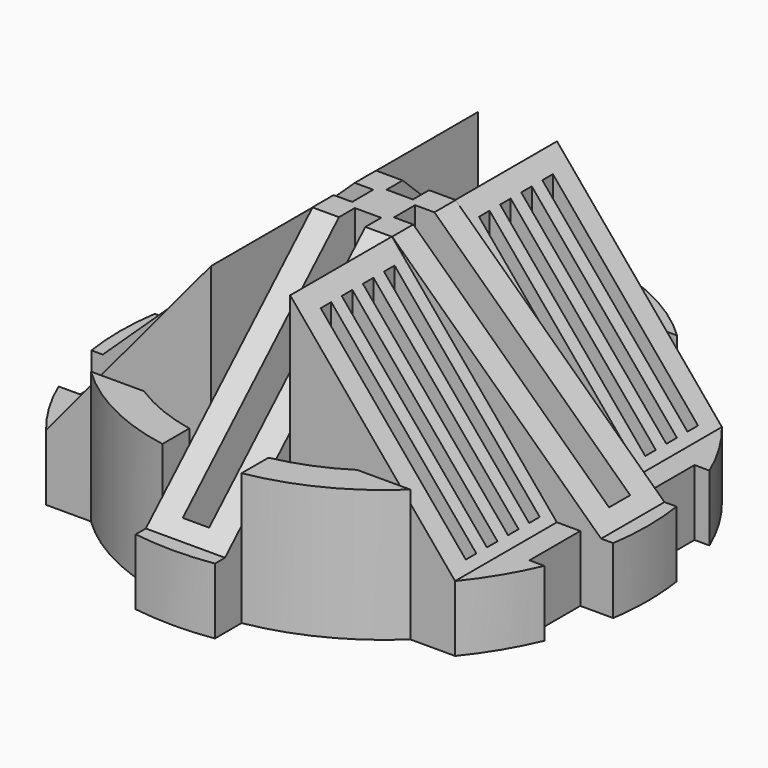
from build123d import *

# Parameters (mm, degrees)
F2_DEPTH  = 12.7
F3_DEPTH  = 25.4
F4_DEPTH  = 38.1
F5_DEPTH  = 50.8
F6_DEPTH  = 50.8
F7_DEPTH  = 50.8
F11_DEPTH = 15.24
F12_DEPTH = 15.24
F13_DEPTH = 15.24
F15_DEPTH = 15.24
F16_W     = 41.402
F16_H     = 5.08
F16_W_2   = 5.08
F16_H_2   = 41.402
F17_DEPTH = 44.45
F18_DEPTH = 50.8
F21_DEPTH = 24.4856
F19_W     = 27.94
F19_H     = 2.54
F22_DEPTH = 44.45
F24_DEPTH = 24.4856
F26_DEPTH = 24.4856
F28_DEPTH = 24.4856
F29_DEPTH = 50.801
F30_DEPTH = 25.4


# Not quite as in the source:
# - after a boolean that leaves OpenCascade's solid faulty, fix() repairs it
# - a feature names something its author has since deleted; it is built from what else it names


with BuildPart() as f2:
    # F1 (on Top) → F2 (new body)
    with BuildSketch(Plane.XY):
        with BuildLine():
            ThreePointArc((50.2252486305, -7.62), (50.6561083702, -3.8208225272), (50.8, 0))
            ThreePointArc((50.8, 0), (50.6561083702, 3.8208225272), (50.2252486305, 7.62))
            Line((50.2252486305, 7.62), (43.8856464383, 7.62))
            Line((43.8856464383, 7.62), (43.8856464383, -7.62))
            Line((43.8856464383, -7.62), (50.2252486305, -7.62))
        make_face()
        with BuildLine():
            Line((43.8856464383, 7.62), (50.2252486305, 7.62))
            ThreePointArc((50.2252486305, 7.62), (48.8754001329, 13.850460709), (46.7558464383, 19.8628))
            Line((46.7558464383, 19.8628), (43.8856464383, 19.8628))
            Line((43.8856464383, 19.8628), (43.8856464383, 7.62))
        make_face()
        with BuildLine():
            ThreePointArc((46.7558464383, -19.8628), (48.8754001329, -13.850460709), (50.2252486305, -7.62))
            Line((50.2252486305, -7.62), (43.8856464383, -7.62))
            Line((43.8856464383, -7.62), (43.8856464383, -19.8628))
            Line((43.8856464383, -19.8628), (46.7558464383, -19.8628))
        make_face()
        with BuildLine():
            Line((43.8856464383, 19.8628), (46.7558464383, 19.8628))
            ThreePointArc((46.7558464383, 19.8628), (43.4950311771, 26.2454236564), (39.3683940318, 32.1056))
            Line((39.3683940318, 32.1056), (30.7413882029, 32.1056))
            ThreePointArc((30.7413882029, 32.1056), (35.7808122406, 26.3730160468), (39.7652068542, 19.8628))
            Line((39.7652068542, 19.8628), (43.8856464383, 19.8628))
        make_face()
        with BuildLine():
            ThreePointArc((39.3683940318, -32.1056), (43.4950311771, -26.2454236564), (46.7558464383, -19.8628))
            Line((46.7558464383, -19.8628), (43.8856464383, -19.8628))
            Line((43.8856464383, -19.8628), (39.7652068542, -19.8628))
            ThreePointArc((39.7652068542, -19.8628), (35.7808122406, -26.3730160468), (30.7413882029, -32.1056))
            Line((30.7413882029, -32.1056), (39.3683940318, -32.1056))
        make_face()
        with BuildLine():
            Line((30.7413882029, 32.1056), (39.3683940318, 32.1056))
            ThreePointArc((39.3683940318, 32.1056), (25.1805025773, 44.1200894146), (7.62, 50.2252486305))
            Line((7.62, 50.2252486305), (7.62, 43.7919867099))
            ThreePointArc((7.62, 43.7919867099), (20.0509833873, 39.670651182), (30.7413882029, 32.1056))
        make_face()
        with BuildLine():
            ThreePointArc((7.62, -50.2252486305), (25.1805025773, -44.1200894146), (39.3683940318, -32.1056))
            Line((39.3683940318, -32.1056), (30.7413882029, -32.1056))
            ThreePointArc((30.7413882029, -32.1056), (20.0509833873, -39.670651182), (7.62, -43.7919867099))
            Line((7.62, -43.7919867099), (7.62, -50.2252486305))
        make_face()
        with BuildLine():
            Line((7.62, 43.7919867099), (7.62, 50.2252486305))
            ThreePointArc((7.62, 50.2252486305), (0, 50.8), (-7.62, 50.2252486305))
            Line((-7.62, 50.2252486305), (-7.62, 43.7919867099))
            ThreePointArc((-7.62, 43.7919867099), (0, 44.45), (7.62, 43.7919867099))
        make_face()
        with BuildLine():
            Line((20.5143961315, 32.1056), (30.7413882029, 32.1056))
            ThreePointArc((30.7413882029, 32.1056), (20.0509833873, 39.670651182), (7.62, 43.7919867099))
            Line((7.62, 43.7919867099), (7.62, 37.33022368))
            ThreePointArc((7.62, 37.33022368), (14.3076984372, 35.3114679025), (20.5143961315, 32.1056))
        make_face()
        with BuildLine():
            ThreePointArc((-7.62, -50.2252486305), (0, -50.8), (7.62, -50.2252486305))
            Line((7.62, -50.2252486305), (7.62, -43.7919867099))
            ThreePointArc((7.62, -43.7919867099), (0, -44.45), (-7.62, -43.7919867099))
            Line((-7.62, -43.7919867099), (-7.62, -50.2252486305))
        make_face()
        with BuildLine():
            ThreePointArc((7.62, -43.7919867099), (20.0509833873, -39.670651182), (30.7413882029, -32.1056))
            Line((30.7413882029, -32.1056), (20.5143961315, -32.1056))
            ThreePointArc((20.5143961315, -32.1056), (14.3076984372, -35.3114679025), (7.62, -37.33022368))
            Line((7.62, -37.33022368), (7.62, -43.7919867099))
        make_face()
        with BuildLine():
            Line((-7.62, 43.7919867099), (-7.62, 50.2252486305))
            ThreePointArc((-7.62, 50.2252486305), (-25.1805025773, 44.1200894146), (-39.3683940318, 32.1056))
            Line((-39.3683940318, 32.1056), (-30.7413882029, 32.1056))
            ThreePointArc((-30.7413882029, 32.1056), (-20.0509833873, 39.670651182), (-7.62, 43.7919867099))
        make_face()
        with BuildLine():
            ThreePointArc((-39.3683940318, -32.1056), (-25.1805025773, -44.1200894146), (-7.62, -50.2252486305))
            Line((-7.62, -50.2252486305), (-7.62, -43.7919867099))
            ThreePointArc((-7.62, -43.7919867099), (-20.0509833873, -39.670651182), (-30.7413882029, -32.1056))
            Line((-30.7413882029, -32.1056), (-39.3683940318, -32.1056))
        make_face()
        with BuildLine():
            Line((-30.7413882029, 32.1056), (-39.3683940318, 32.1056))
            ThreePointArc((-39.3683940318, 32.1056), (-43.4950311771, 26.2454236564), (-46.7558464383, 19.8628))
            Line((-46.7558464383, 19.8628), (-42.6407977939, 19.8628))
            Line((-42.6407977939, 19.8628), (-39.7652068542, 19.8628))
            ThreePointArc((-39.7652068542, 19.8628), (-35.7808122406, 26.3730160468), (-30.7413882029, 32.1056))
        make_face()
        with BuildLine():
            Line((-7.62, 37.33022368), (-7.62, 43.7919867099))
            ThreePointArc((-7.62, 43.7919867099), (-20.0509833873, 39.670651182), (-30.7413882029, 32.1056))
            Line((-30.7413882029, 32.1056), (-20.5143961315, 32.1056))
            ThreePointArc((-20.5143961315, 32.1056), (-14.3076984372, 35.3114679025), (-7.62, 37.33022368))
        make_face()
        with BuildLine():
            ThreePointArc((-46.7558464383, -19.8628), (-43.4950311771, -26.2454236564), (-39.3683940318, -32.1056))
            Line((-39.3683940318, -32.1056), (-30.7413882029, -32.1056))
            ThreePointArc((-30.7413882029, -32.1056), (-35.7808122406, -26.3730160468), (-39.7652068542, -19.8628))
            Line((-39.7652068542, -19.8628), (-42.6407977939, -19.8628))
            Line((-42.6407977939, -19.8628), (-46.7558464383, -19.8628))
        make_face()
        with BuildLine():
            ThreePointArc((-30.7413882029, -32.1056), (-20.0509833873, -39.670651182), (-7.62, -43.7919867099))
            Line((-7.62, -43.7919867099), (-7.62, -37.33022368))
            ThreePointArc((-7.62, -37.33022368), (-14.2009349705, -35.3545392554), (-20.32, -32.2289869527))
            ThreePointArc((-20.32, -32.2289869527), (-20.4172912734, -32.1674403249), (-20.5143961315, -32.1056))
            Line((-20.5143961315, -32.1056), (-30.7413882029, -32.1056))
        make_face()
        with BuildLine():
            Line((-42.6407977939, 19.8628), (-46.7558464383, 19.8628))
            ThreePointArc((-46.7558464383, 19.8628), (-48.8754001329, 13.850460709), (-50.2252486305, 7.62))
            Line((-50.2252486305, 7.62), (-42.6407977939, 7.62))
            Line((-42.6407977939, 7.62), (-42.6407977939, 19.8628))
        make_face()
        with BuildLine():
            ThreePointArc((-50.2252486305, -7.62), (-48.8754001329, -13.850460709), (-46.7558464383, -19.8628))
            Line((-46.7558464383, -19.8628), (-42.6407977939, -19.8628))
            Line((-42.6407977939, -19.8628), (-42.6407977939, -7.62))
            Line((-42.6407977939, -7.62), (-50.2252486305, -7.62))
        make_face()
        with BuildLine():
            Line((-42.6407977939, 7.62), (-50.2252486305, 7.62))
            ThreePointArc((-50.2252486305, 7.62), (-50.8, 0), (-50.2252486305, -7.62))
            Line((-50.2252486305, -7.62), (-42.6407977939, -7.62))
            Line((-42.6407977939, -7.62), (-42.6407977939, 7.62))
        make_face()
    extrude(amount=F2_DEPTH)

    # F1 (on Top) → F3 (join)
    with BuildSketch(Plane.XY):
        with BuildLine():
            ThreePointArc((-30.7413882029, -32.1056), (-20.0509833873, -39.670651182), (-7.62, -43.7919867099))
            Line((-7.62, -43.7919867099), (-7.62, -37.33022368))
            ThreePointArc((-7.62, -37.33022368), (-14.2009349705, -35.3545392554), (-20.32, -32.2289869527))
            ThreePointArc((-20.32, -32.2289869527), (-20.4172912734, -32.1674403249), (-20.5143961315, -32.1056))
            Line((-20.5143961315, -32.1056), (-30.7413882029, -32.1056))
        make_face()
        with BuildLine():
            ThreePointArc((7.62, -43.7919867099), (20.0509833873, -39.670651182), (30.7413882029, -32.1056))
            Line((30.7413882029, -32.1056), (20.5143961315, -32.1056))
            ThreePointArc((20.5143961315, -32.1056), (14.3076984372, -35.3114679025), (7.62, -37.33022368))
            Line((7.62, -37.33022368), (7.62, -43.7919867099))
        make_face()
        with BuildLine():
            Line((20.5143961315, -32.1056), (30.7413882029, -32.1056))
            ThreePointArc((30.7413882029, -32.1056), (35.7808122406, -26.3730160468), (39.7652068542, -19.8628))
            Line((39.7652068542, -19.8628), (32.5127540538, -19.8628))
            ThreePointArc((32.5127540538, -19.8628), (27.2110492659, -26.667748271), (20.5143961315, -32.1056))
        make_face()
        with BuildLine():
            Line((7.62, 37.33022368), (7.62, 43.7919867099))
            ThreePointArc((7.62, 43.7919867099), (0, 44.45), (-7.62, 43.7919867099))
            Line((-7.62, 43.7919867099), (-7.62, 37.33022368))
            ThreePointArc((-7.62, 37.33022368), (0, 38.1), (7.62, 37.33022368))
        make_face()
        with BuildLine():
            ThreePointArc((-7.62, -43.7919867099), (0, -44.45), (7.62, -43.7919867099))
            Line((7.62, -43.7919867099), (7.62, -37.33022368))
            ThreePointArc((7.62, -37.33022368), (0, -38.1), (-7.62, -37.33022368))
            Line((-7.62, -37.33022368), (-7.62, -43.7919867099))
        make_face()
        with BuildLine():
            Line((-37.33022368, 7.62), (-42.6407977939, 7.62))
            Line((-42.6407977939, 7.62), (-42.6407977939, -7.62))
            Line((-42.6407977939, -7.62), (-37.33022368, -7.62))
            ThreePointArc((-37.33022368, -7.62), (-38.1, 0), (-37.33022368, 7.62))
        make_face()
        with BuildLine():
            Line((-42.6407977939, -7.62), (-42.6407977939, -19.8628))
            Line((-42.6407977939, -19.8628), (-39.7652068542, -19.8628))
            Line((-39.7652068542, -19.8628), (-32.5127540538, -19.8628))
            ThreePointArc((-32.5127540538, -19.8628), (-35.4539408619, -13.9509167211), (-37.33022368, -7.62))
            Line((-37.33022368, -7.62), (-42.6407977939, -7.62))
        make_face()
        with BuildLine():
            ThreePointArc((-39.7652068542, -19.8628), (-35.7808122406, -26.3730160468), (-30.7413882029, -32.1056))
            Line((-30.7413882029, -32.1056), (-20.5143961315, -32.1056))
            ThreePointArc((-20.5143961315, -32.1056), (-27.2110492659, -26.667748271), (-32.5127540538, -19.8628))
            Line((-32.5127540538, -19.8628), (-39.7652068542, -19.8628))
        make_face()
        with BuildLine():
            Line((-39.7652068542, 19.8628), (-42.6407977939, 19.8628))
            Line((-42.6407977939, 19.8628), (-42.6407977939, 7.62))
            Line((-42.6407977939, 7.62), (-37.33022368, 7.62))
            ThreePointArc((-37.33022368, 7.62), (-35.4539408619, 13.9509167211), (-32.5127540538, 19.8628))
            Line((-32.5127540538, 19.8628), (-39.7652068542, 19.8628))
        make_face()
        with BuildLine():
            Line((-20.5143961315, 32.1056), (-30.7413882029, 32.1056))
            ThreePointArc((-30.7413882029, 32.1056), (-35.7808122406, 26.3730160468), (-39.7652068542, 19.8628))
            Line((-39.7652068542, 19.8628), (-32.5127540538, 19.8628))
            ThreePointArc((-32.5127540538, 19.8628), (-27.2110492659, 26.667748271), (-20.5143961315, 32.1056))
        make_face()
        with BuildLine():
            Line((-7.62, 37.33022368), (-7.62, 43.7919867099))
            ThreePointArc((-7.62, 43.7919867099), (-20.0509833873, 39.670651182), (-30.7413882029, 32.1056))
            Line((-30.7413882029, 32.1056), (-20.5143961315, 32.1056))
            ThreePointArc((-20.5143961315, 32.1056), (-14.3076984372, 35.3114679025), (-7.62, 37.33022368))
        make_face()
        with BuildLine():
            ThreePointArc((39.7652068542, 19.8628), (35.7808122406, 26.3730160468), (30.7413882029, 32.1056))
            Line((30.7413882029, 32.1056), (20.5143961315, 32.1056))
            ThreePointArc((20.5143961315, 32.1056), (27.2110492659, 26.667748271), (32.5127540538, 19.8628))
            Line((32.5127540538, 19.8628), (39.7652068542, 19.8628))
        make_face()
        with BuildLine():
            Line((37.33022368, 7.62), (43.8856464383, 7.62))
            Line((43.8856464383, 7.62), (43.8856464383, 19.8628))
            Line((43.8856464383, 19.8628), (39.7652068542, 19.8628))
            Line((39.7652068542, 19.8628), (32.5127540538, 19.8628))
            ThreePointArc((32.5127540538, 19.8628), (35.4539408619, 13.9509167211), (37.33022368, 7.62))
        make_face()
        with BuildLine():
            Line((43.8856464383, -19.8628), (43.8856464383, -7.62))
            Line((43.8856464383, -7.62), (37.33022368, -7.62))
            ThreePointArc((37.33022368, -7.62), (35.4539408619, -13.9509167211), (32.5127540538, -19.8628))
            Line((32.5127540538, -19.8628), (39.7652068542, -19.8628))
            Line((39.7652068542, -19.8628), (43.8856464383, -19.8628))
        make_face()
        with BuildLine():
            Line((43.8856464383, -7.62), (43.8856464383, 7.62))
            Line((43.8856464383, 7.62), (37.33022368, 7.62))
            ThreePointArc((37.33022368, 7.62), (38.1, 0), (37.33022368, -7.62))
            Line((37.33022368, -7.62), (43.8856464383, -7.62))
        make_face()
        with BuildLine():
            Line((20.5143961315, 32.1056), (30.7413882029, 32.1056))
            ThreePointArc((30.7413882029, 32.1056), (20.0509833873, 39.670651182), (7.62, 43.7919867099))
            Line((7.62, 43.7919867099), (7.62, 37.33022368))
            ThreePointArc((7.62, 37.33022368), (14.3076984372, 35.3114679025), (20.5143961315, 32.1056))
        make_face()
    extrude(amount=F3_DEPTH)

    # F1 (on Top) → F4 (join)
    with BuildSketch(Plane.XY):
        with BuildLine():
            ThreePointArc((-7.62, -37.33022368), (0, -38.1), (7.62, -37.33022368))
            Line((7.62, -37.33022368), (7.62, -32.1056))
            Line((7.62, -32.1056), (7.62, -30.8220391928))
            ThreePointArc((7.62, -30.8220391928), (0, -31.75), (-7.62, -30.8220391928))
            Line((-7.62, -30.8220391928), (-7.62, -32.1056))
            Line((-7.62, -32.1056), (-7.62, -37.33022368))
        make_face()
        with BuildLine():
            Line((-7.62, 32.1056), (-7.62, 37.33022368))
            ThreePointArc((-7.62, 37.33022368), (-14.3076984372, 35.3114679025), (-20.5143961315, 32.1056))
            Line((-20.5143961315, 32.1056), (-7.62, 32.1056))
        make_face()
        with BuildLine():
            ThreePointArc((-24.769571578, 19.8628), (-17.0967048776, 26.7537881865), (-7.62, 30.8220391928))
            Line((-7.62, 30.8220391928), (-7.62, 32.1056))
            Line((-7.62, 32.1056), (-20.5143961315, 32.1056))
            ThreePointArc((-20.5143961315, 32.1056), (-27.2110492659, 26.667748271), (-32.5127540538, 19.8628))
            Line((-32.5127540538, 19.8628), (-24.769571578, 19.8628))
        make_face()
        with BuildLine():
            ThreePointArc((-30.8220391928, 7.62), (-28.4618751136, 14.0706845966), (-24.769571578, 19.8628))
            Line((-24.769571578, 19.8628), (-32.5127540538, 19.8628))
            ThreePointArc((-32.5127540538, 19.8628), (-35.4539408619, 13.9509167211), (-37.33022368, 7.62))
            Line((-37.33022368, 7.62), (-30.8220391928, 7.62))
        make_face()
        with BuildLine():
            ThreePointArc((-30.8220391928, -7.62), (-31.75, 0), (-30.8220391928, 7.62))
            Line((-30.8220391928, 7.62), (-37.33022368, 7.62))
            ThreePointArc((-37.33022368, 7.62), (-38.1, 0), (-37.33022368, -7.62))
            Line((-37.33022368, -7.62), (-30.8220391928, -7.62))
        make_face()
        with BuildLine():
            Line((-32.5127540538, -19.8628), (-24.769571578, -19.8628))
            ThreePointArc((-24.769571578, -19.8628), (-28.4618751136, -14.0706845966), (-30.8220391928, -7.62))
            Line((-30.8220391928, -7.62), (-37.33022368, -7.62))
            ThreePointArc((-37.33022368, -7.62), (-35.4539408619, -13.9509167211), (-32.5127540538, -19.8628))
        make_face()
        with BuildLine():
            Line((-7.62, -32.1056), (-7.62, -30.8220391928))
            ThreePointArc((-7.62, -30.8220391928), (-17.0967048776, -26.7537881865), (-24.769571578, -19.8628))
            Line((-24.769571578, -19.8628), (-32.5127540538, -19.8628))
            ThreePointArc((-32.5127540538, -19.8628), (-27.2110492659, -26.667748271), (-20.5143961315, -32.1056))
            Line((-20.5143961315, -32.1056), (-20.32, -32.1056))
            Line((-20.32, -32.1056), (-7.62, -32.1056))
        make_face()
        with BuildLine():
            Line((-20.32, -32.1056), (-20.5143961315, -32.1056))
            ThreePointArc((-20.5143961315, -32.1056), (-20.4172912734, -32.1674403249), (-20.32, -32.2289869527))
            Line((-20.32, -32.2289869527), (-20.32, -32.1056))
        make_face()
        with BuildLine():
            ThreePointArc((-20.32, -32.2289869527), (-14.2009349705, -35.3545392554), (-7.62, -37.33022368))
            Line((-7.62, -37.33022368), (-7.62, -32.1056))
            Line((-7.62, -32.1056), (-20.32, -32.1056))
            Line((-20.32, -32.1056), (-20.32, -32.2289869527))
        make_face()
        with BuildLine():
            ThreePointArc((7.62, -37.33022368), (14.3076984372, -35.3114679025), (20.5143961315, -32.1056))
            Line((20.5143961315, -32.1056), (7.62, -32.1056))
            Line((7.62, -32.1056), (7.62, -37.33022368))
        make_face()
        with BuildLine():
            ThreePointArc((20.5143961315, -32.1056), (27.2110492659, -26.667748271), (32.5127540538, -19.8628))
            Line((32.5127540538, -19.8628), (24.769571578, -19.8628))
            ThreePointArc((24.769571578, -19.8628), (17.0967048776, -26.7537881865), (7.62, -30.8220391928))
            Line((7.62, -30.8220391928), (7.62, -32.1056))
            Line((7.62, -32.1056), (20.5143961315, -32.1056))
        make_face()
        with BuildLine():
            ThreePointArc((32.5127540538, -19.8628), (35.4539408619, -13.9509167211), (37.33022368, -7.62))
            Line((37.33022368, -7.62), (30.8220391928, -7.62))
            ThreePointArc((30.8220391928, -7.62), (28.4618751136, -14.0706845966), (24.769571578, -19.8628))
            Line((24.769571578, -19.8628), (32.5127540538, -19.8628))
        make_face()
        with BuildLine():
            ThreePointArc((37.33022368, -7.62), (38.1, 0), (37.33022368, 7.62))
            Line((37.33022368, 7.62), (30.8220391928, 7.62))
            ThreePointArc((30.8220391928, 7.62), (31.5171559977, 3.8381477062), (31.75, 0))
            ThreePointArc((31.75, 0), (31.5171559977, -3.8381477062), (30.8220391928, -7.62))
            Line((30.8220391928, -7.62), (37.33022368, -7.62))
        make_face()
        with BuildLine():
            Line((30.8220391928, 7.62), (37.33022368, 7.62))
            ThreePointArc((37.33022368, 7.62), (35.4539408619, 13.9509167211), (32.5127540538, 19.8628))
            Line((32.5127540538, 19.8628), (24.769571578, 19.8628))
            ThreePointArc((24.769571578, 19.8628), (28.4618751136, 14.0706845966), (30.8220391928, 7.62))
        make_face()
        with BuildLine():
            Line((24.769571578, 19.8628), (32.5127540538, 19.8628))
            ThreePointArc((32.5127540538, 19.8628), (27.2110492659, 26.667748271), (20.5143961315, 32.1056))
            Line((20.5143961315, 32.1056), (7.62, 32.1056))
            Line((7.62, 32.1056), (7.62, 30.8220391928))
            ThreePointArc((7.62, 30.8220391928), (17.0967048776, 26.7537881865), (24.769571578, 19.8628))
        make_face()
        with BuildLine():
            Line((7.62, 32.1056), (20.5143961315, 32.1056))
            ThreePointArc((20.5143961315, 32.1056), (14.3076984372, 35.3114679025), (7.62, 37.33022368))
            Line((7.62, 37.33022368), (7.62, 32.1056))
        make_face()
        with BuildLine():
            Line((7.62, 32.1056), (7.62, 37.33022368))
            ThreePointArc((7.62, 37.33022368), (0, 38.1), (-7.62, 37.33022368))
            Line((-7.62, 37.33022368), (-7.62, 32.1056))
            Line((-7.62, 32.1056), (-7.62, 30.8220391928))
            ThreePointArc((-7.62, 30.8220391928), (0, 31.75), (7.62, 30.8220391928))
            Line((7.62, 30.8220391928), (7.62, 32.1056))
        make_face()
    extrude(amount=F4_DEPTH)

    # F1 (on Top) → F5 (join)
    with BuildSketch(Plane.XY):
        with BuildLine():
            Line((7.62, 24.230055716), (7.62, 30.8220391928))
            ThreePointArc((7.62, 30.8220391928), (0, 31.75), (-7.62, 30.8220391928))
            Line((-7.62, 30.8220391928), (-7.62, 24.230055716))
            ThreePointArc((-7.62, 24.230055716), (0, 25.4), (7.62, 24.230055716))
        make_face()
        with BuildLine():
            ThreePointArc((-7.62, -30.8220391928), (0, -31.75), (7.62, -30.8220391928))
            Line((7.62, -30.8220391928), (7.62, -24.230055716))
            ThreePointArc((7.62, -24.230055716), (0, -25.4), (-7.62, -24.230055716))
            Line((-7.62, -24.230055716), (-7.62, -30.8220391928))
        make_face()
        with BuildLine():
            ThreePointArc((7.62, -30.8220391928), (17.0967048776, -26.7537881865), (24.769571578, -19.8628))
            Line((24.769571578, -19.8628), (15.8312720954, -19.8628))
            ThreePointArc((15.8312720954, -19.8628), (11.9272281502, -22.4254593856), (7.62, -24.230055716))
            Line((7.62, -24.230055716), (7.62, -30.8220391928))
        make_face()
        with BuildLine():
            Line((15.8312720954, 19.8628), (24.769571578, 19.8628))
            ThreePointArc((24.769571578, 19.8628), (17.0967048776, 26.7537881865), (7.62, 30.8220391928))
            Line((7.62, 30.8220391928), (7.62, 24.230055716))
            ThreePointArc((7.62, 24.230055716), (11.9272281502, 22.4254593856), (15.8312720954, 19.8628))
        make_face()
        with BuildLine():
            Line((-24.230055716, 7.62), (-30.8220391928, 7.62))
            ThreePointArc((-30.8220391928, 7.62), (-31.75, 0), (-30.8220391928, -7.62))
            Line((-30.8220391928, -7.62), (-24.230055716, -7.62))
            ThreePointArc((-24.230055716, -7.62), (-25.4, 0), (-24.230055716, 7.62))
        make_face()
        with BuildLine():
            Line((-7.62, 24.230055716), (-7.62, 30.8220391928))
            ThreePointArc((-7.62, 30.8220391928), (-17.0967048776, 26.7537881865), (-24.769571578, 19.8628))
            Line((-24.769571578, 19.8628), (-15.8312720954, 19.8628))
            ThreePointArc((-15.8312720954, 19.8628), (-11.9272281502, 22.4254593856), (-7.62, 24.230055716))
        make_face()
        with BuildLine():
            ThreePointArc((31.75, 0), (31.5171559977, 3.8381477062), (30.8220391928, 7.62))
            Line((30.8220391928, 7.62), (24.230055716, 7.62))
            ThreePointArc((24.230055716, 7.62), (25.1058102357, 3.8546455618), (25.4, 0))
            ThreePointArc((25.4, 0), (25.1058102357, -3.8546455618), (24.230055716, -7.62))
            Line((24.230055716, -7.62), (30.8220391928, -7.62))
            ThreePointArc((30.8220391928, -7.62), (31.5171559977, -3.8381477062), (31.75, 0))
        make_face()
        with BuildLine():
            ThreePointArc((-24.769571578, -19.8628), (-17.0967048776, -26.7537881865), (-7.62, -30.8220391928))
            Line((-7.62, -30.8220391928), (-7.62, -24.230055716))
            ThreePointArc((-7.62, -24.230055716), (-11.9272281502, -22.4254593856), (-15.8312720954, -19.8628))
            Line((-15.8312720954, -19.8628), (-20.32, -19.8628))
            Line((-20.32, -19.8628), (-24.769571578, -19.8628))
        make_face()
        with BuildLine():
            ThreePointArc((-30.8220391928, -7.62), (-28.4618751136, -14.0706845966), (-24.769571578, -19.8628))
            Line((-24.769571578, -19.8628), (-20.32, -19.8628))
            Line((-20.32, -19.8628), (-15.8312720954, -19.8628))
            ThreePointArc((-15.8312720954, -19.8628), (-20.9451434577, -14.3687496163), (-24.230055716, -7.62))
            Line((-24.230055716, -7.62), (-30.8220391928, -7.62))
        make_face()
    extrude(amount=F5_DEPTH)



with BuildPart() as f2b:
    # F1 (on Top) → F2, piece 2 (new body)
    with BuildSketch(Plane.XY):
        Polygon((2.54, 7.62), (7.62, 7.62), (7.62, 17.78), (0, 10.16), align=None)
        Polygon((7.62, 2.54), (7.62, 7.62), (2.54, 7.62), align=None)
    extrude(amount=F2_DEPTH)


with BuildPart() as f2c:
    # F1 (on Top) → F2, piece 3 (new body)
    with BuildSketch(Plane.XY):
        Polygon((2.54, -7.62), (7.62, -7.62), (7.62, -2.54), align=None)
    extrude(amount=F2_DEPTH)


with BuildPart() as f2d:
    # F1 (on Top) → F2, piece 4 (new body)
    with BuildSketch(Plane.XY):
        Polygon((-7.62, -17.78), (0, -10.16), (-2.54, -7.62), (-7.62, -7.62), align=None)
    extrude(amount=F2_DEPTH)


with BuildPart() as f2e:
    # F1 (on Top) → F2, piece 5 (new body)
    with BuildSketch(Plane.XY):
        Polygon((-7.62, 2.54), (-2.54, 7.62), (-7.62, 7.62), align=None)
    extrude(amount=F2_DEPTH)


with BuildPart() as f2_1:
    add(f2.part)

    add(f2b.part)  # F6 merges F2b

    add(f2c.part)  # F6 merges F2c

    add(f2d.part)  # F6 merges F2d

    add(f2e.part)  # F6 merges F2e
    # F1 (on Top) → F6 (join)
    with BuildSketch(Plane.XY):
        with BuildLine():
            ThreePointArc((-7.62, -50.2252486305), (0, -50.8), (7.62, -50.2252486305))
            Line((7.62, -50.2252486305), (7.62, -43.7919867099))
            ThreePointArc((7.62, -43.7919867099), (0, -44.45), (-7.62, -43.7919867099))
            Line((-7.62, -43.7919867099), (-7.62, -50.2252486305))
        make_face()
        with BuildLine():
            ThreePointArc((-7.62, -37.33022368), (0, -38.1), (7.62, -37.33022368))
            Line((7.62, -37.33022368), (7.62, -32.1056))
            Line((7.62, -32.1056), (7.62, -30.8220391928))
            ThreePointArc((7.62, -30.8220391928), (0, -31.75), (-7.62, -30.8220391928))
            Line((-7.62, -30.8220391928), (-7.62, -32.1056))
            Line((-7.62, -32.1056), (-7.62, -37.33022368))
        make_face()
        with BuildLine():
            ThreePointArc((-7.62, -30.8220391928), (0, -31.75), (7.62, -30.8220391928))
            Line((7.62, -30.8220391928), (7.62, -24.230055716))
            ThreePointArc((7.62, -24.230055716), (0, -25.4), (-7.62, -24.230055716))
            Line((-7.62, -24.230055716), (-7.62, -30.8220391928))
        make_face()
        with BuildLine():
            ThreePointArc((-7.62, -43.7919867099), (0, -44.45), (7.62, -43.7919867099))
            Line((7.62, -43.7919867099), (7.62, -37.33022368))
            ThreePointArc((7.62, -37.33022368), (0, -38.1), (-7.62, -37.33022368))
            Line((-7.62, -37.33022368), (-7.62, -43.7919867099))
        make_face()
        with BuildLine():
            ThreePointArc((-7.62, -24.230055716), (0, -25.4), (7.62, -24.230055716))
            Line((7.62, -24.230055716), (7.62, -19.8628))
            Line((7.62, -19.8628), (7.62, -17.78))
            Line((7.62, -17.78), (0, -10.16))
            Line((0, -10.16), (-7.62, -17.78))
            Line((-7.62, -17.78), (-7.62, -19.8628))
            Line((-7.62, -19.8628), (-7.62, -24.230055716))
        make_face()
        with BuildLine():
            Line((7.62, 19.8628), (7.62, 24.230055716))
            ThreePointArc((7.62, 24.230055716), (0, 25.4), (-7.62, 24.230055716))
            Line((-7.62, 24.230055716), (-7.62, 19.8628))
            Line((-7.62, 19.8628), (-7.62, 17.78))
            Line((-7.62, 17.78), (0, 10.16))
            Line((0, 10.16), (7.62, 17.78))
            Line((7.62, 17.78), (7.62, 19.8628))
        make_face()
        with BuildLine():
            Line((7.62, 24.230055716), (7.62, 30.8220391928))
            ThreePointArc((7.62, 30.8220391928), (0, 31.75), (-7.62, 30.8220391928))
            Line((-7.62, 30.8220391928), (-7.62, 24.230055716))
            ThreePointArc((-7.62, 24.230055716), (0, 25.4), (7.62, 24.230055716))
        make_face()
        with BuildLine():
            Line((7.62, 32.1056), (7.62, 37.33022368))
            ThreePointArc((7.62, 37.33022368), (0, 38.1), (-7.62, 37.33022368))
            Line((-7.62, 37.33022368), (-7.62, 32.1056))
            Line((-7.62, 32.1056), (-7.62, 30.8220391928))
            ThreePointArc((-7.62, 30.8220391928), (0, 31.75), (7.62, 30.8220391928))
            Line((7.62, 30.8220391928), (7.62, 32.1056))
        make_face()
        with BuildLine():
            Line((7.62, 37.33022368), (7.62, 43.7919867099))
            ThreePointArc((7.62, 43.7919867099), (0, 44.45), (-7.62, 43.7919867099))
            Line((-7.62, 43.7919867099), (-7.62, 37.33022368))
            ThreePointArc((-7.62, 37.33022368), (0, 38.1), (7.62, 37.33022368))
        make_face()
        with BuildLine():
            Line((7.62, 43.7919867099), (7.62, 50.2252486305))
            ThreePointArc((7.62, 50.2252486305), (0, 50.8), (-7.62, 50.2252486305))
            Line((-7.62, 50.2252486305), (-7.62, 43.7919867099))
            ThreePointArc((-7.62, 43.7919867099), (0, 44.45), (7.62, 43.7919867099))
        make_face()
        Polygon((7.62, -17.78), (7.62, -7.62), (2.54, -7.62), (0, -10.16), align=None)
        Polygon((-2.54, 7.62), (0, 10.16), (-7.62, 17.78), (-7.62, 7.62), align=None)
        Polygon((-7.62, -7.62), (-2.54, -7.62), (-7.62, -2.54), align=None)
        Polygon((-7.62, -17.78), (0, -10.16), (-2.54, -7.62), (-7.62, -7.62), align=None)
        Polygon((7.62, -2.54), (7.62, 2.54), (2.54, 7.62), (0, 7.62), (-2.54, 7.62), (-7.62, 2.54), (-7.62, -2.54), (-2.54, -7.62), (0, -7.62), (2.54, -7.62), align=None)
        Polygon((2.54, 7.62), (7.62, 7.62), (7.62, 17.78), (0, 10.16), align=None)
        Polygon((0, 7.62), (2.54, 7.62), (0, 10.16), (-2.54, 7.62), align=None)
        Polygon((0, -10.16), (2.54, -7.62), (0, -7.62), (-2.54, -7.62), align=None)
        Polygon((-7.62, 2.54), (-2.54, 7.62), (-7.62, 7.62), align=None)
        Polygon((2.54, -7.62), (7.62, -7.62), (7.62, -2.54), align=None)
        Polygon((7.62, 2.54), (7.62, 7.62), (2.54, 7.62), align=None)
    extrude(amount=F6_DEPTH)

    # F1 (on Top) → F7 (join)
    with BuildSketch(Plane.XY):
        with BuildLine():
            ThreePointArc((-24.230055716, -7.62), (-20.9451434577, -14.3687496163), (-15.8312720954, -19.8628))
            Line((-15.8312720954, -19.8628), (-7.62, -19.8628))
            Line((-7.62, -19.8628), (-7.62, -17.78))
            Line((-7.62, -17.78), (-7.62, -7.62))
            Line((-7.62, -7.62), (-17.78, -7.62))
            Line((-17.78, -7.62), (-24.230055716, -7.62))
        make_face()
        with BuildLine():
            ThreePointArc((-15.8312720954, -19.8628), (-11.9272281502, -22.4254593856), (-7.62, -24.230055716))
            Line((-7.62, -24.230055716), (-7.62, -19.8628))
            Line((-7.62, -19.8628), (-15.8312720954, -19.8628))
        make_face()
        with BuildLine():
            Line((-42.6407977939, 7.62), (-50.2252486305, 7.62))
            ThreePointArc((-50.2252486305, 7.62), (-50.8, 0), (-50.2252486305, -7.62))
            Line((-50.2252486305, -7.62), (-42.6407977939, -7.62))
            Line((-42.6407977939, -7.62), (-42.6407977939, 7.62))
        make_face()
        with BuildLine():
            Line((-37.33022368, 7.62), (-42.6407977939, 7.62))
            Line((-42.6407977939, 7.62), (-42.6407977939, -7.62))
            Line((-42.6407977939, -7.62), (-37.33022368, -7.62))
            ThreePointArc((-37.33022368, -7.62), (-38.1, 0), (-37.33022368, 7.62))
        make_face()
        with BuildLine():
            ThreePointArc((-30.8220391928, -7.62), (-31.75, 0), (-30.8220391928, 7.62))
            Line((-30.8220391928, 7.62), (-37.33022368, 7.62))
            ThreePointArc((-37.33022368, 7.62), (-38.1, 0), (-37.33022368, -7.62))
            Line((-37.33022368, -7.62), (-30.8220391928, -7.62))
        make_face()
        with BuildLine():
            Line((-24.230055716, 7.62), (-30.8220391928, 7.62))
            ThreePointArc((-30.8220391928, 7.62), (-31.75, 0), (-30.8220391928, -7.62))
            Line((-30.8220391928, -7.62), (-24.230055716, -7.62))
            ThreePointArc((-24.230055716, -7.62), (-25.4, 0), (-24.230055716, 7.62))
        make_face()
        with BuildLine():
            Line((-17.78, 7.62), (-24.230055716, 7.62))
            ThreePointArc((-24.230055716, 7.62), (-25.4, 0), (-24.230055716, -7.62))
            Line((-24.230055716, -7.62), (-17.78, -7.62))
            Line((-17.78, -7.62), (-10.16, 0))
            Line((-10.16, 0), (-17.78, 7.62))
        make_face()
        Polygon((-7.62, -7.62), (-2.54, -7.62), (-7.62, -2.54), align=None)
        with BuildLine():
            ThreePointArc((25.4, 0), (25.1058102357, 3.8546455618), (24.230055716, 7.62))
            Line((24.230055716, 7.62), (17.78, 7.62))
            Line((17.78, 7.62), (10.16, 0))
            Line((10.16, 0), (17.78, -7.62))
            Line((17.78, -7.62), (24.230055716, -7.62))
            ThreePointArc((24.230055716, -7.62), (25.1058102357, -3.8546455618), (25.4, 0))
        make_face()
        with BuildLine():
            ThreePointArc((31.75, 0), (31.5171559977, 3.8381477062), (30.8220391928, 7.62))
            Line((30.8220391928, 7.62), (24.230055716, 7.62))
            ThreePointArc((24.230055716, 7.62), (25.1058102357, 3.8546455618), (25.4, 0))
            ThreePointArc((25.4, 0), (25.1058102357, -3.8546455618), (24.230055716, -7.62))
            Line((24.230055716, -7.62), (30.8220391928, -7.62))
            ThreePointArc((30.8220391928, -7.62), (31.5171559977, -3.8381477062), (31.75, 0))
        make_face()
        with BuildLine():
            ThreePointArc((37.33022368, -7.62), (38.1, 0), (37.33022368, 7.62))
            Line((37.33022368, 7.62), (30.8220391928, 7.62))
            ThreePointArc((30.8220391928, 7.62), (31.5171559977, 3.8381477062), (31.75, 0))
            ThreePointArc((31.75, 0), (31.5171559977, -3.8381477062), (30.8220391928, -7.62))
            Line((30.8220391928, -7.62), (37.33022368, -7.62))
        make_face()
        with BuildLine():
            ThreePointArc((50.2252486305, -7.62), (50.6561083702, -3.8208225272), (50.8, 0))
            ThreePointArc((50.8, 0), (50.6561083702, 3.8208225272), (50.2252486305, 7.62))
            Line((50.2252486305, 7.62), (43.8856464383, 7.62))
            Line((43.8856464383, 7.62), (43.8856464383, -7.62))
            Line((43.8856464383, -7.62), (50.2252486305, -7.62))
        make_face()
        Polygon((-10.16, 0), (-17.78, -7.62), (-7.62, -7.62), (-7.62, -2.54), align=None)
        Polygon((10.16, 0), (17.78, 7.62), (7.62, 7.62), (7.62, 2.54), align=None)
        Polygon((-7.62, -2.54), (-7.62, 2.54), (-10.16, 0), align=None)
        Polygon((7.62, -2.54), (10.16, 0), (7.62, 2.54), align=None)
        Polygon((-7.62, 7.62), (-17.78, 7.62), (-10.16, 0), (-7.62, 2.54), align=None)
        Polygon((7.62, -7.62), (17.78, -7.62), (10.16, 0), (7.62, -2.54), align=None)
        with BuildLine():
            ThreePointArc((15.8312720954, -19.8628), (20.9451434577, -14.3687496163), (24.230055716, -7.62))
            Line((24.230055716, -7.62), (17.78, -7.62))
            Line((17.78, -7.62), (7.62, -7.62))
            Line((7.62, -7.62), (7.62, -17.78))
            Line((7.62, -17.78), (7.62, -19.8628))
            Line((7.62, -19.8628), (15.8312720954, -19.8628))
        make_face()
        with BuildLine():
            Line((17.78, 7.62), (24.230055716, 7.62))
            ThreePointArc((24.230055716, 7.62), (20.9451434577, 14.3687496163), (15.8312720954, 19.8628))
            Line((15.8312720954, 19.8628), (7.62, 19.8628))
            Line((7.62, 19.8628), (7.62, 17.78))
            Line((7.62, 17.78), (7.62, 7.62))
            Line((7.62, 7.62), (17.78, 7.62))
        make_face()
        with BuildLine():
            Line((-7.62, 19.8628), (-15.8312720954, 19.8628))
            ThreePointArc((-15.8312720954, 19.8628), (-20.9451434577, 14.3687496163), (-24.230055716, 7.62))
            Line((-24.230055716, 7.62), (-17.78, 7.62))
            Line((-17.78, 7.62), (-7.62, 7.62))
            Line((-7.62, 7.62), (-7.62, 17.78))
            Line((-7.62, 17.78), (-7.62, 19.8628))
        make_face()
        with BuildLine():
            Line((43.8856464383, -7.62), (43.8856464383, 7.62))
            Line((43.8856464383, 7.62), (37.33022368, 7.62))
            ThreePointArc((37.33022368, 7.62), (38.1, 0), (37.33022368, -7.62))
            Line((37.33022368, -7.62), (43.8856464383, -7.62))
        make_face()
    extrude(amount=F7_DEPTH)

    # F8 (on face) → F11 (cut)
    with BuildSketch(Plane.XZ.offset(7.62)):
        Polygon((-55.5124618113, 12.7), (-48.0377227068, 12.7), (-7.6606776565, 50.8), (-7.6606776565, 65.3503203437), (-55.9246055782, 65.3503203437), align=None)
    extrude(amount=-F11_DEPTH, mode=Mode.SUBTRACT)

    # F9 (on face) → F12 (cut)
    with BuildSketch(Plane.XZ.offset(7.62)):
        Polygon((7.6703908853, 50.8), (47.8966571391, 12.7), (55.3924329579, 12.7), (55.3924329579, 55.8396019042), (7.6703908853, 53.9275594056), align=None)
    extrude(amount=-F12_DEPTH, mode=Mode.SUBTRACT)

    # F10 (on face) → F13 (cut)
    with BuildSketch(Plane.YZ.offset(7.62)):
        Polygon((-58.5949867964, 12.7), (-47.7943047881, 12.7), (-7.6625170186, 50.8), (-7.6625170186, 52.6358112693), (-57.5197674334, 52.6358112693), align=None)
    extrude(amount=-F13_DEPTH, mode=Mode.SUBTRACT)

    # F14 (on face) → F15 (cut)
    with BuildSketch(Plane(origin=(-7.62, 0, 0), x_dir=(0, -1, 0), z_dir=(-1, 0, 0))):
        Polygon((-54.0386848152, 12.7), (-47.7350726724, 12.7), (-7.6549332589, 50.8), (-7.6549332589, 52.5853484869), (-58.2393705845, 53.2422102988), align=None)
    extrude(amount=-F15_DEPTH, mode=Mode.SUBTRACT)

    # F16 (on offset) → F17 (cut)
    with BuildSketch(Plane.XY.offset(50.8)):
        with Locations((24.6556571391, 0)):
            Rectangle(F16_W, F16_H)
        with Locations((-24.7967227068, 0)):
            Rectangle(F16_W, F16_H)
        with Locations((0, 24.4940726724)):
            Rectangle(F16_W_2, F16_H_2)
        with Locations((0, -24.5533047881)):
            Rectangle(F16_W_2, F16_H_2)
    extrude(amount=-F17_DEPTH, mode=Mode.SUBTRACT)

    # F1 (on Top) → F18 (join)
    with BuildSketch(Plane.XY):
        with BuildLine():
            ThreePointArc((-24.230055716, -7.62), (-20.9451434577, -14.3687496163), (-15.8312720954, -19.8628))
            Line((-15.8312720954, -19.8628), (-7.62, -19.8628))
            Line((-7.62, -19.8628), (-7.62, -17.78))
            Line((-7.62, -17.78), (-7.62, -7.62))
            Line((-7.62, -7.62), (-17.78, -7.62))
            Line((-17.78, -7.62), (-24.230055716, -7.62))
        make_face()
        with BuildLine():
            ThreePointArc((-30.8220391928, -7.62), (-28.4618751136, -14.0706845966), (-24.769571578, -19.8628))
            Line((-24.769571578, -19.8628), (-20.32, -19.8628))
            Line((-20.32, -19.8628), (-15.8312720954, -19.8628))
            ThreePointArc((-15.8312720954, -19.8628), (-20.9451434577, -14.3687496163), (-24.230055716, -7.62))
            Line((-24.230055716, -7.62), (-30.8220391928, -7.62))
        make_face()
        with BuildLine():
            Line((-32.5127540538, -19.8628), (-24.769571578, -19.8628))
            ThreePointArc((-24.769571578, -19.8628), (-28.4618751136, -14.0706845966), (-30.8220391928, -7.62))
            Line((-30.8220391928, -7.62), (-37.33022368, -7.62))
            ThreePointArc((-37.33022368, -7.62), (-35.4539408619, -13.9509167211), (-32.5127540538, -19.8628))
        make_face()
        with BuildLine():
            Line((-42.6407977939, -7.62), (-42.6407977939, -19.8628))
            Line((-42.6407977939, -19.8628), (-39.7652068542, -19.8628))
            Line((-39.7652068542, -19.8628), (-32.5127540538, -19.8628))
            ThreePointArc((-32.5127540538, -19.8628), (-35.4539408619, -13.9509167211), (-37.33022368, -7.62))
            Line((-37.33022368, -7.62), (-42.6407977939, -7.62))
        make_face()
        with BuildLine():
            ThreePointArc((-50.2252486305, -7.62), (-48.8754001329, -13.850460709), (-46.7558464383, -19.8628))
            Line((-46.7558464383, -19.8628), (-42.6407977939, -19.8628))
            Line((-42.6407977939, -19.8628), (-42.6407977939, -7.62))
            Line((-42.6407977939, -7.62), (-50.2252486305, -7.62))
        make_face()
        with BuildLine():
            ThreePointArc((-15.8312720954, -19.8628), (-11.9272281502, -22.4254593856), (-7.62, -24.230055716))
            Line((-7.62, -24.230055716), (-7.62, -19.8628))
            Line((-7.62, -19.8628), (-15.8312720954, -19.8628))
        make_face()
        with BuildLine():
            ThreePointArc((-24.769571578, -19.8628), (-17.0967048776, -26.7537881865), (-7.62, -30.8220391928))
            Line((-7.62, -30.8220391928), (-7.62, -24.230055716))
            ThreePointArc((-7.62, -24.230055716), (-11.9272281502, -22.4254593856), (-15.8312720954, -19.8628))
            Line((-15.8312720954, -19.8628), (-20.32, -19.8628))
            Line((-20.32, -19.8628), (-24.769571578, -19.8628))
        make_face()
        with BuildLine():
            Line((-7.62, -32.1056), (-7.62, -30.8220391928))
            ThreePointArc((-7.62, -30.8220391928), (-17.0967048776, -26.7537881865), (-24.769571578, -19.8628))
            Line((-24.769571578, -19.8628), (-32.5127540538, -19.8628))
            ThreePointArc((-32.5127540538, -19.8628), (-27.2110492659, -26.667748271), (-20.5143961315, -32.1056))
            Line((-20.5143961315, -32.1056), (-20.32, -32.1056))
            Line((-20.32, -32.1056), (-7.62, -32.1056))
        make_face()
        with BuildLine():
            ThreePointArc((-39.7652068542, -19.8628), (-35.7808122406, -26.3730160468), (-30.7413882029, -32.1056))
            Line((-30.7413882029, -32.1056), (-20.5143961315, -32.1056))
            ThreePointArc((-20.5143961315, -32.1056), (-27.2110492659, -26.667748271), (-32.5127540538, -19.8628))
            Line((-32.5127540538, -19.8628), (-39.7652068542, -19.8628))
        make_face()
        with BuildLine():
            ThreePointArc((-46.7558464383, -19.8628), (-43.4950311771, -26.2454236564), (-39.3683940318, -32.1056))
            Line((-39.3683940318, -32.1056), (-30.7413882029, -32.1056))
            ThreePointArc((-30.7413882029, -32.1056), (-35.7808122406, -26.3730160468), (-39.7652068542, -19.8628))
            Line((-39.7652068542, -19.8628), (-42.6407977939, -19.8628))
            Line((-42.6407977939, -19.8628), (-46.7558464383, -19.8628))
        make_face()
        with BuildLine():
            Line((-30.7413882029, 32.1056), (-39.3683940318, 32.1056))
            ThreePointArc((-39.3683940318, 32.1056), (-43.4950311771, 26.2454236564), (-46.7558464383, 19.8628))
            Line((-46.7558464383, 19.8628), (-42.6407977939, 19.8628))
            Line((-42.6407977939, 19.8628), (-39.7652068542, 19.8628))
            ThreePointArc((-39.7652068542, 19.8628), (-35.7808122406, 26.3730160468), (-30.7413882029, 32.1056))
        make_face()
        with BuildLine():
            Line((-42.6407977939, 19.8628), (-46.7558464383, 19.8628))
            ThreePointArc((-46.7558464383, 19.8628), (-48.8754001329, 13.850460709), (-50.2252486305, 7.62))
            Line((-50.2252486305, 7.62), (-42.6407977939, 7.62))
            Line((-42.6407977939, 7.62), (-42.6407977939, 19.8628))
        make_face()
        with BuildLine():
            Line((-20.5143961315, 32.1056), (-30.7413882029, 32.1056))
            ThreePointArc((-30.7413882029, 32.1056), (-35.7808122406, 26.3730160468), (-39.7652068542, 19.8628))
            Line((-39.7652068542, 19.8628), (-32.5127540538, 19.8628))
            ThreePointArc((-32.5127540538, 19.8628), (-27.2110492659, 26.667748271), (-20.5143961315, 32.1056))
        make_face()
        with BuildLine():
            Line((-39.7652068542, 19.8628), (-42.6407977939, 19.8628))
            Line((-42.6407977939, 19.8628), (-42.6407977939, 7.62))
            Line((-42.6407977939, 7.62), (-37.33022368, 7.62))
            ThreePointArc((-37.33022368, 7.62), (-35.4539408619, 13.9509167211), (-32.5127540538, 19.8628))
            Line((-32.5127540538, 19.8628), (-39.7652068542, 19.8628))
        make_face()
        with BuildLine():
            ThreePointArc((-24.769571578, 19.8628), (-17.0967048776, 26.7537881865), (-7.62, 30.8220391928))
            Line((-7.62, 30.8220391928), (-7.62, 32.1056))
            Line((-7.62, 32.1056), (-20.5143961315, 32.1056))
            ThreePointArc((-20.5143961315, 32.1056), (-27.2110492659, 26.667748271), (-32.5127540538, 19.8628))
            Line((-32.5127540538, 19.8628), (-24.769571578, 19.8628))
        make_face()
        with BuildLine():
            ThreePointArc((-30.8220391928, 7.62), (-28.4618751136, 14.0706845966), (-24.769571578, 19.8628))
            Line((-24.769571578, 19.8628), (-32.5127540538, 19.8628))
            ThreePointArc((-32.5127540538, 19.8628), (-35.4539408619, 13.9509167211), (-37.33022368, 7.62))
            Line((-37.33022368, 7.62), (-30.8220391928, 7.62))
        make_face()
        with BuildLine():
            Line((-7.62, 24.230055716), (-7.62, 30.8220391928))
            ThreePointArc((-7.62, 30.8220391928), (-17.0967048776, 26.7537881865), (-24.769571578, 19.8628))
            Line((-24.769571578, 19.8628), (-15.8312720954, 19.8628))
            ThreePointArc((-15.8312720954, 19.8628), (-11.9272281502, 22.4254593856), (-7.62, 24.230055716))
        make_face()
        with BuildLine():
            Line((-15.8312720954, 19.8628), (-24.769571578, 19.8628))
            ThreePointArc((-24.769571578, 19.8628), (-28.4618751136, 14.0706845966), (-30.8220391928, 7.62))
            Line((-30.8220391928, 7.62), (-24.230055716, 7.62))
            ThreePointArc((-24.230055716, 7.62), (-20.9451434577, 14.3687496163), (-15.8312720954, 19.8628))
        make_face()
        with BuildLine():
            Line((-7.62, 19.8628), (-15.8312720954, 19.8628))
            ThreePointArc((-15.8312720954, 19.8628), (-20.9451434577, 14.3687496163), (-24.230055716, 7.62))
            Line((-24.230055716, 7.62), (-17.78, 7.62))
            Line((-17.78, 7.62), (-7.62, 7.62))
            Line((-7.62, 7.62), (-7.62, 17.78))
            Line((-7.62, 17.78), (-7.62, 19.8628))
        make_face()
        with BuildLine():
            Line((-7.62, 19.8628), (-7.62, 24.230055716))
            ThreePointArc((-7.62, 24.230055716), (-11.9272281502, 22.4254593856), (-15.8312720954, 19.8628))
            Line((-15.8312720954, 19.8628), (-7.62, 19.8628))
        make_face()
        with BuildLine():
            ThreePointArc((7.62, -24.230055716), (11.9272281502, -22.4254593856), (15.8312720954, -19.8628))
            Line((15.8312720954, -19.8628), (7.62, -19.8628))
            Line((7.62, -19.8628), (7.62, -24.230055716))
        make_face()
        with BuildLine():
            ThreePointArc((7.62, -30.8220391928), (17.0967048776, -26.7537881865), (24.769571578, -19.8628))
            Line((24.769571578, -19.8628), (15.8312720954, -19.8628))
            ThreePointArc((15.8312720954, -19.8628), (11.9272281502, -22.4254593856), (7.62, -24.230055716))
            Line((7.62, -24.230055716), (7.62, -30.8220391928))
        make_face()
        with BuildLine():
            Line((20.5143961315, -32.1056), (30.7413882029, -32.1056))
            ThreePointArc((30.7413882029, -32.1056), (35.7808122406, -26.3730160468), (39.7652068542, -19.8628))
            Line((39.7652068542, -19.8628), (32.5127540538, -19.8628))
            ThreePointArc((32.5127540538, -19.8628), (27.2110492659, -26.667748271), (20.5143961315, -32.1056))
        make_face()
        with BuildLine():
            ThreePointArc((20.5143961315, -32.1056), (27.2110492659, -26.667748271), (32.5127540538, -19.8628))
            Line((32.5127540538, -19.8628), (24.769571578, -19.8628))
            ThreePointArc((24.769571578, -19.8628), (17.0967048776, -26.7537881865), (7.62, -30.8220391928))
            Line((7.62, -30.8220391928), (7.62, -32.1056))
            Line((7.62, -32.1056), (20.5143961315, -32.1056))
        make_face()
        with BuildLine():
            ThreePointArc((39.3683940318, -32.1056), (43.4950311771, -26.2454236564), (46.7558464383, -19.8628))
            Line((46.7558464383, -19.8628), (43.8856464383, -19.8628))
            Line((43.8856464383, -19.8628), (39.7652068542, -19.8628))
            ThreePointArc((39.7652068542, -19.8628), (35.7808122406, -26.3730160468), (30.7413882029, -32.1056))
            Line((30.7413882029, -32.1056), (39.3683940318, -32.1056))
        make_face()
        with BuildLine():
            ThreePointArc((15.8312720954, -19.8628), (20.9451434577, -14.3687496163), (24.230055716, -7.62))
            Line((24.230055716, -7.62), (17.78, -7.62))
            Line((17.78, -7.62), (7.62, -7.62))
            Line((7.62, -7.62), (7.62, -17.78))
            Line((7.62, -17.78), (7.62, -19.8628))
            Line((7.62, -19.8628), (15.8312720954, -19.8628))
        make_face()
        with BuildLine():
            ThreePointArc((24.769571578, -19.8628), (28.4618751136, -14.0706845966), (30.8220391928, -7.62))
            Line((30.8220391928, -7.62), (24.230055716, -7.62))
            ThreePointArc((24.230055716, -7.62), (20.9451434577, -14.3687496163), (15.8312720954, -19.8628))
            Line((15.8312720954, -19.8628), (24.769571578, -19.8628))
        make_face()
        with BuildLine():
            ThreePointArc((32.5127540538, -19.8628), (35.4539408619, -13.9509167211), (37.33022368, -7.62))
            Line((37.33022368, -7.62), (30.8220391928, -7.62))
            ThreePointArc((30.8220391928, -7.62), (28.4618751136, -14.0706845966), (24.769571578, -19.8628))
            Line((24.769571578, -19.8628), (32.5127540538, -19.8628))
        make_face()
        with BuildLine():
            ThreePointArc((46.7558464383, -19.8628), (48.8754001329, -13.850460709), (50.2252486305, -7.62))
            Line((50.2252486305, -7.62), (43.8856464383, -7.62))
            Line((43.8856464383, -7.62), (43.8856464383, -19.8628))
            Line((43.8856464383, -19.8628), (46.7558464383, -19.8628))
        make_face()
        with BuildLine():
            Line((17.78, 7.62), (24.230055716, 7.62))
            ThreePointArc((24.230055716, 7.62), (20.9451434577, 14.3687496163), (15.8312720954, 19.8628))
            Line((15.8312720954, 19.8628), (7.62, 19.8628))
            Line((7.62, 19.8628), (7.62, 17.78))
            Line((7.62, 17.78), (7.62, 7.62))
            Line((7.62, 7.62), (17.78, 7.62))
        make_face()
        with BuildLine():
            Line((24.230055716, 7.62), (30.8220391928, 7.62))
            ThreePointArc((30.8220391928, 7.62), (28.4618751136, 14.0706845966), (24.769571578, 19.8628))
            Line((24.769571578, 19.8628), (15.8312720954, 19.8628))
            ThreePointArc((15.8312720954, 19.8628), (20.9451434577, 14.3687496163), (24.230055716, 7.62))
        make_face()
        with BuildLine():
            Line((30.8220391928, 7.62), (37.33022368, 7.62))
            ThreePointArc((37.33022368, 7.62), (35.4539408619, 13.9509167211), (32.5127540538, 19.8628))
            Line((32.5127540538, 19.8628), (24.769571578, 19.8628))
            ThreePointArc((24.769571578, 19.8628), (28.4618751136, 14.0706845966), (30.8220391928, 7.62))
        make_face()
        with BuildLine():
            Line((43.8856464383, 7.62), (50.2252486305, 7.62))
            ThreePointArc((50.2252486305, 7.62), (48.8754001329, 13.850460709), (46.7558464383, 19.8628))
            Line((46.7558464383, 19.8628), (43.8856464383, 19.8628))
            Line((43.8856464383, 19.8628), (43.8856464383, 7.62))
        make_face()
        with BuildLine():
            Line((43.8856464383, 19.8628), (46.7558464383, 19.8628))
            ThreePointArc((46.7558464383, 19.8628), (43.4950311771, 26.2454236564), (39.3683940318, 32.1056))
            Line((39.3683940318, 32.1056), (30.7413882029, 32.1056))
            ThreePointArc((30.7413882029, 32.1056), (35.7808122406, 26.3730160468), (39.7652068542, 19.8628))
            Line((39.7652068542, 19.8628), (43.8856464383, 19.8628))
        make_face()
        with BuildLine():
            Line((24.769571578, 19.8628), (32.5127540538, 19.8628))
            ThreePointArc((32.5127540538, 19.8628), (27.2110492659, 26.667748271), (20.5143961315, 32.1056))
            Line((20.5143961315, 32.1056), (7.62, 32.1056))
            Line((7.62, 32.1056), (7.62, 30.8220391928))
            ThreePointArc((7.62, 30.8220391928), (17.0967048776, 26.7537881865), (24.769571578, 19.8628))
        make_face()
        with BuildLine():
            Line((15.8312720954, 19.8628), (24.769571578, 19.8628))
            ThreePointArc((24.769571578, 19.8628), (17.0967048776, 26.7537881865), (7.62, 30.8220391928))
            Line((7.62, 30.8220391928), (7.62, 24.230055716))
            ThreePointArc((7.62, 24.230055716), (11.9272281502, 22.4254593856), (15.8312720954, 19.8628))
        make_face()
        with BuildLine():
            Line((7.62, 19.8628), (15.8312720954, 19.8628))
            ThreePointArc((15.8312720954, 19.8628), (11.9272281502, 22.4254593856), (7.62, 24.230055716))
            Line((7.62, 24.230055716), (7.62, 19.8628))
        make_face()
        with BuildLine():
            ThreePointArc((39.7652068542, 19.8628), (35.7808122406, 26.3730160468), (30.7413882029, 32.1056))
            Line((30.7413882029, 32.1056), (20.5143961315, 32.1056))
            ThreePointArc((20.5143961315, 32.1056), (27.2110492659, 26.667748271), (32.5127540538, 19.8628))
            Line((32.5127540538, 19.8628), (39.7652068542, 19.8628))
        make_face()
        with BuildLine():
            Line((37.33022368, 7.62), (43.8856464383, 7.62))
            Line((43.8856464383, 7.62), (43.8856464383, 19.8628))
            Line((43.8856464383, 19.8628), (39.7652068542, 19.8628))
            Line((39.7652068542, 19.8628), (32.5127540538, 19.8628))
            ThreePointArc((32.5127540538, 19.8628), (35.4539408619, 13.9509167211), (37.33022368, 7.62))
        make_face()
        with BuildLine():
            Line((43.8856464383, -19.8628), (43.8856464383, -7.62))
            Line((43.8856464383, -7.62), (37.33022368, -7.62))
            ThreePointArc((37.33022368, -7.62), (35.4539408619, -13.9509167211), (32.5127540538, -19.8628))
            Line((32.5127540538, -19.8628), (39.7652068542, -19.8628))
            Line((39.7652068542, -19.8628), (43.8856464383, -19.8628))
        make_face()
    extrude(amount=F18_DEPTH)

    # F20 (on face) → F21 (cut)
    with BuildSketch(Plane.XZ.offset(32.1056)):
        Polygon((-39.3683940318, 12.7), (-7.62, 50.8), (-7.62, 65.6115189195), (-60.1087734103, 65.6115189195), (-60.1087734103, 12.7), align=None)
    extrude(amount=-F21_DEPTH, mode=Mode.SUBTRACT)

    # F19 (on offset) → F22 (cut)
    with BuildSketch(Plane.XY.offset(50.8)):
        with Locations((-24.13, -11.43)):
            Rectangle(F19_W, F19_H)
        with Locations((-24.13, -16.51)):
            Rectangle(F19_W, F19_H)
        with Locations((-24.13, 11.43)):
            Rectangle(F19_W, F19_H)
        with Locations((-24.13, 16.51)):
            Rectangle(F19_W, F19_H)
        with Locations((24.13, 16.51)):
            Rectangle(F19_W, F19_H)
        with Locations((24.13, 11.43)):
            Rectangle(F19_W, F19_H)
        with Locations((24.13, -11.43)):
            Rectangle(F19_W, F19_H)
        with Locations((24.13, -16.51)):
            Rectangle(F19_W, F19_H)
        with Locations((-24.13, 21.59)):
            Rectangle(F19_W, F19_H)
        with Locations((-24.13, 26.67)):
            Rectangle(F19_W, F19_H)
        with Locations((-24.13, -21.59)):
            Rectangle(F19_W, F19_H)
        with Locations((-24.13, -26.67)):
            Rectangle(F19_W, F19_H)
        with Locations((24.13, -21.59)):
            Rectangle(F19_W, F19_H)
        with Locations((24.13, -26.67)):
            Rectangle(F19_W, F19_H)
        with Locations((24.13, 21.59)):
            Rectangle(F19_W, F19_H)
        with Locations((24.13, 26.67)):
            Rectangle(F19_W, F19_H)
    extrude(amount=-F22_DEPTH, mode=Mode.SUBTRACT)

    # F23 (on face) → F24 (cut)
    with BuildSketch(Plane(origin=(0, 32.1056, 0), x_dir=(-1, 0, 0), z_dir=(0, 1, 0))):
        Polygon((7.62, 58.9498654008), (7.62, 50.8), (39.3683940318, 12.7), (63.3994191885, 12.7), (63.3994191885, 58.9498654008), align=None)
    extrude(amount=-F24_DEPTH, mode=Mode.SUBTRACT)

    # F25 (on face) → F26 (cut)
    with BuildSketch(Plane(origin=(0, 32.1056, 0), x_dir=(-1, 0, 0), z_dir=(0, 1, 0))):
        Polygon((-39.3683940318, 12.7), (-7.62, 50.8), (-7.62, 60.825034976), (-64.4157677889, 60.825034976), (-64.4157677889, 12.7), align=None)
    extrude(amount=-F26_DEPTH, mode=Mode.SUBTRACT)

    # F27 (on face) → F28 (cut)
    with BuildSketch(Plane.XZ.offset(32.1056)):
        Polygon((7.62, 58.3216398954), (7.62, 50.8), (39.3683940318, 12.7), (79.0987238288, 12.7), (79.0987238288, 63.607044518), align=None)
    extrude(amount=-F28_DEPTH, mode=Mode.SUBTRACT)

    # F1 (on Top) → F29 (cut, through all)
    with BuildSketch(Plane.XY):
        with BuildLine():
            ThreePointArc((-20.32, -32.2289869527), (-14.2009349705, -35.3545392554), (-7.62, -37.33022368))
            Line((-7.62, -37.33022368), (-7.62, -32.1056))
            Line((-7.62, -32.1056), (-20.32, -32.1056))
            Line((-20.32, -32.1056), (-20.32, -32.2289869527))
        make_face()
        with BuildLine():
            Line((-20.32, -32.1056), (-20.5143961315, -32.1056))
            ThreePointArc((-20.5143961315, -32.1056), (-20.4172912734, -32.1674403249), (-20.32, -32.2289869527))
            Line((-20.32, -32.2289869527), (-20.32, -32.1056))
        make_face()
        with BuildLine():
            ThreePointArc((7.62, -37.33022368), (14.3076984372, -35.3114679025), (20.5143961315, -32.1056))
            Line((20.5143961315, -32.1056), (7.62, -32.1056))
            Line((7.62, -32.1056), (7.62, -37.33022368))
        make_face()
        with BuildLine():
            Line((7.62, 32.1056), (20.5143961315, 32.1056))
            ThreePointArc((20.5143961315, 32.1056), (14.3076984372, 35.3114679025), (7.62, 37.33022368))
            Line((7.62, 37.33022368), (7.62, 32.1056))
        make_face()
        with BuildLine():
            Line((-7.62, 32.1056), (-7.62, 37.33022368))
            ThreePointArc((-7.62, 37.33022368), (-14.3076984372, 35.3114679025), (-20.5143961315, 32.1056))
            Line((-20.5143961315, 32.1056), (-7.62, 32.1056))
        make_face()
        with BuildLine():
            Line((-42.6407977939, 19.8628), (-46.7558464383, 19.8628))
            ThreePointArc((-46.7558464383, 19.8628), (-48.8754001329, 13.850460709), (-50.2252486305, 7.62))
            Line((-50.2252486305, 7.62), (-42.6407977939, 7.62))
            Line((-42.6407977939, 7.62), (-42.6407977939, 19.8628))
        make_face()
        with BuildLine():
            ThreePointArc((-50.2252486305, -7.62), (-48.8754001329, -13.850460709), (-46.7558464383, -19.8628))
            Line((-46.7558464383, -19.8628), (-42.6407977939, -19.8628))
            Line((-42.6407977939, -19.8628), (-42.6407977939, -7.62))
            Line((-42.6407977939, -7.62), (-50.2252486305, -7.62))
        make_face()
        with BuildLine():
            ThreePointArc((46.7558464383, -19.8628), (48.8754001329, -13.850460709), (50.2252486305, -7.62))
            Line((50.2252486305, -7.62), (43.8856464383, -7.62))
            Line((43.8856464383, -7.62), (43.8856464383, -19.8628))
            Line((43.8856464383, -19.8628), (46.7558464383, -19.8628))
        make_face()
        with BuildLine():
            Line((43.8856464383, 7.62), (50.2252486305, 7.62))
            ThreePointArc((50.2252486305, 7.62), (48.8754001329, 13.850460709), (46.7558464383, 19.8628))
            Line((46.7558464383, 19.8628), (43.8856464383, 19.8628))
            Line((43.8856464383, 19.8628), (43.8856464383, 7.62))
        make_face()
    extrude(amount=F29_DEPTH, mode=Mode.SUBTRACT)

    # F1 (on Top) → F30 (cut)
    with BuildSketch(Plane.XY):
        with BuildLine():
            Line((30.7413882029, 32.1056), (39.3683940318, 32.1056))
            ThreePointArc((39.3683940318, 32.1056), (25.1805025773, 44.1200894146), (7.62, 50.2252486305))
            Line((7.62, 50.2252486305), (7.62, 43.7919867099))
            ThreePointArc((7.62, 43.7919867099), (20.0509833873, 39.670651182), (30.7413882029, 32.1056))
        make_face()
        with BuildLine():
            Line((-7.62, 43.7919867099), (-7.62, 50.2252486305))
            ThreePointArc((-7.62, 50.2252486305), (-25.1805025773, 44.1200894146), (-39.3683940318, 32.1056))
            Line((-39.3683940318, 32.1056), (-30.7413882029, 32.1056))
            ThreePointArc((-30.7413882029, 32.1056), (-20.0509833873, 39.670651182), (-7.62, 43.7919867099))
        make_face()
        with BuildLine():
            ThreePointArc((-39.3683940318, -32.1056), (-25.1805025773, -44.1200894146), (-7.62, -50.2252486305))
            Line((-7.62, -50.2252486305), (-7.62, -43.7919867099))
            ThreePointArc((-7.62, -43.7919867099), (-20.0509833873, -39.670651182), (-30.7413882029, -32.1056))
            Line((-30.7413882029, -32.1056), (-39.3683940318, -32.1056))
        make_face()
        with BuildLine():
            ThreePointArc((7.62, -50.2252486305), (25.1805025773, -44.1200894146), (39.3683940318, -32.1056))
            Line((39.3683940318, -32.1056), (30.7413882029, -32.1056))
            ThreePointArc((30.7413882029, -32.1056), (20.0509833873, -39.670651182), (7.62, -43.7919867099))
            Line((7.62, -43.7919867099), (7.62, -50.2252486305))
        make_face()
    extrude(amount=F30_DEPTH, mode=Mode.SUBTRACT)

    add(f2_1.part.fix(), mode=Mode.REPLACE)


solid = f2_1.part
